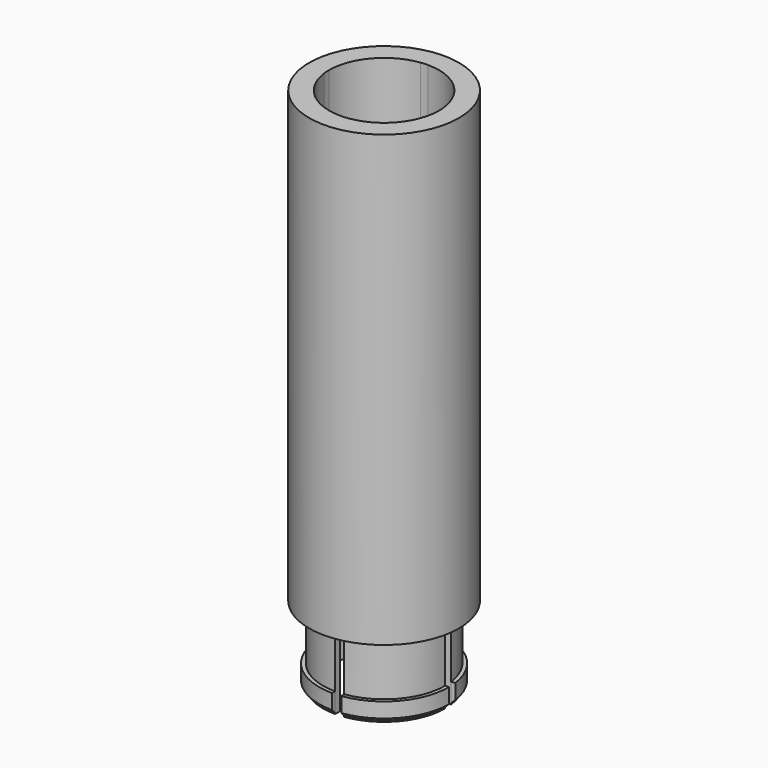
from build123d import *
from build123d import SkipClean  # not in build123d's __all__

# Parameters (mm, degrees)
F0_R          = 15
F1_DEPTH      = 90
F2_DEPTH      = 15
F3_START      = -11
F3_DEPTH      = 4
F4_T2_ANGLE   = 105.003910896
F4_2_T2_ANGLE = 105.003910896
F4_3_T2_ANGLE = 105.003910896
F4_4_T2_ANGLE = 105.003910896


# Not quite as in the source:
# - a fillet or chamfer that OpenCascade refuses, or shapes differently, is made with other operations: its cross-section is extruded or revolved along the edge and cut away or added


with BuildPart() as f1:
    # F0 (on Top) → F1 (new body)
    with BuildSketch(Plane.XY):
        with Locations((-39.9452038109, 28.1051583588)):
            Circle(F0_R)
        with BuildLine():
            ThreePointArc((-27.061585061, 29.8407758013), (-26.9743317556, 28.9749158684), (-26.9452038109, 28.1051583588))
            ThreePointArc((-26.9452038109, 28.1051583588), (-30.1584007897, 19.5483782036), (-38.2095863684, 15.2215396089))
            ThreePointArc((-38.2095863684, 15.2215396089), (-39.0754463013, 15.1342863035), (-39.9452038109, 15.1051583588))
            ThreePointArc((-39.9452038109, 15.1051583588), (-48.5019839661, 18.3183553376), (-52.8288225609, 26.3695409163))
            ThreePointArc((-52.8288225609, 26.3695409163), (-52.9160758662, 27.2354008492), (-52.9452038109, 28.1051583588))
            ThreePointArc((-52.9452038109, 28.1051583588), (-49.7320068322, 36.661938514), (-41.6808212534, 40.9887771087))
            ThreePointArc((-41.6808212534, 40.9887771087), (-40.8149613205, 41.0760304141), (-39.9452038109, 41.1051583588))
            ThreePointArc((-39.9452038109, 41.1051583588), (-31.3884236558, 37.89196138), (-27.061585061, 29.8407758013))
        make_face(mode=Mode.SUBTRACT)
        with BuildLine():
            ThreePointArc((-52.0855368637, 26.4696726918), (-48.0083235725, 18.8829785888), (-39.9452038109, 15.8551583588))
            Line((-39.9452038109, 15.8551583588), (-39.9452038109, 17.1051583588))
            ThreePointArc((-39.9452038109, 17.1051583588), (-47.1855562499, 19.8240173409), (-50.8467273686, 26.6365589844))
            Line((-50.8467273686, 26.6365589844), (-52.0855368637, 26.4696726918))
        make_face()
        with BuildLine():
            ThreePointArc((-27.8048707581, 29.7406440258), (-27.7226512973, 28.9247375506), (-27.6952038109, 28.1051583588))
            Line((-27.6952038109, 28.1051583588), (-26.9452038109, 28.1051583588))
            ThreePointArc((-26.9452038109, 28.1051583588), (-26.9743317556, 28.9749158684), (-27.061585061, 29.8407758013))
            Line((-27.061585061, 29.8407758013), (-27.8048707581, 29.7406440258))
        make_face()
        with BuildLine():
            ThreePointArc((-39.9452038109, 40.3551583588), (-31.8820840493, 37.3273381288), (-27.8048707581, 29.7406440258))
            Line((-27.8048707581, 29.7406440258), (-27.061585061, 29.8407758013))
            ThreePointArc((-27.061585061, 29.8407758013), (-31.3884236558, 37.89196138), (-39.9452038109, 41.1051583588))
            Line((-39.9452038109, 41.1051583588), (-39.9452038109, 40.3551583588))
        make_face()
        with BuildLine():
            ThreePointArc((-41.5806894779, 40.2454914116), (-40.7647830027, 40.3277108724), (-39.9452038109, 40.3551583588))
            Line((-39.9452038109, 40.3551583588), (-39.9452038109, 41.1051583588))
            ThreePointArc((-39.9452038109, 41.1051583588), (-40.8149613205, 41.0760304141), (-41.6808212534, 40.9887771087))
            Line((-41.6808212534, 40.9887771087), (-41.5806894779, 40.2454914116))
        make_face()
        with BuildLine():
            ThreePointArc((-52.1952038109, 28.1051583588), (-49.1673835809, 36.1682781204), (-41.5806894779, 40.2454914116))
            Line((-41.5806894779, 40.2454914116), (-41.6808212534, 40.9887771087))
            ThreePointArc((-41.6808212534, 40.9887771087), (-49.7320068322, 36.661938514), (-52.9452038109, 28.1051583588))
            Line((-52.9452038109, 28.1051583588), (-52.1952038109, 28.1051583588))
        make_face()
        with BuildLine():
            Line((-52.8288225609, 26.3695409163), (-52.0855368637, 26.4696726918))
            ThreePointArc((-52.0855368637, 26.4696726918), (-52.1677563246, 27.2855791671), (-52.1952038109, 28.1051583588))
            Line((-52.1952038109, 28.1051583588), (-52.9452038109, 28.1051583588))
            ThreePointArc((-52.9452038109, 28.1051583588), (-52.9160758662, 27.2354008492), (-52.8288225609, 26.3695409163))
        make_face()
        with BuildLine():
            Line((-39.9452038109, 15.1051583588), (-39.9452038109, 15.8551583588))
            ThreePointArc((-39.9452038109, 15.8551583588), (-48.0083235725, 18.8829785888), (-52.0855368637, 26.4696726918))
            Line((-52.0855368637, 26.4696726918), (-52.8288225609, 26.3695409163))
            ThreePointArc((-52.8288225609, 26.3695409163), (-48.5019839661, 18.3183553376), (-39.9452038109, 15.1051583588))
        make_face()
        with BuildLine():
            Line((-38.2095863684, 15.2215396089), (-38.309718144, 15.964825306))
            ThreePointArc((-38.309718144, 15.964825306), (-39.1256246192, 15.8826058452), (-39.9452038109, 15.8551583588))
            Line((-39.9452038109, 15.8551583588), (-39.9452038109, 15.1051583588))
            ThreePointArc((-39.9452038109, 15.1051583588), (-39.0754463013, 15.1342863035), (-38.2095863684, 15.2215396089))
        make_face()
        with BuildLine():
            Line((-26.9452038109, 28.1051583588), (-27.6952038109, 28.1051583588))
            ThreePointArc((-27.6952038109, 28.1051583588), (-30.7230240409, 20.0420385972), (-38.309718144, 15.964825306))
            Line((-38.309718144, 15.964825306), (-38.2095863684, 15.2215396089))
            ThreePointArc((-38.2095863684, 15.2215396089), (-30.1584007897, 19.5483782036), (-26.9452038109, 28.1051583588))
        make_face()
        with BuildLine():
            ThreePointArc((-38.309718144, 15.964825306), (-30.7230240409, 20.0420385972), (-27.6952038109, 28.1051583588))
            Line((-27.6952038109, 28.1051583588), (-28.9452038109, 28.1051583588))
            ThreePointArc((-28.9452038109, 28.1051583588), (-31.664062793, 20.8648059198), (-38.4766044365, 17.2036348012))
            Line((-38.4766044365, 17.2036348012), (-38.309718144, 15.964825306))
        make_face()
        with BuildLine():
            Line((-29.0436802533, 29.5737577332), (-27.8048707581, 29.7406440258))
            ThreePointArc((-27.8048707581, 29.7406440258), (-31.8820840493, 37.3273381288), (-39.9452038109, 40.3551583588))
            Line((-39.9452038109, 40.3551583588), (-39.9452038109, 39.1051583588))
            ThreePointArc((-39.9452038109, 39.1051583588), (-32.7048513719, 36.3862993768), (-29.0436802533, 29.5737577332))
        make_face()
        with BuildLine():
            Line((-41.4138031853, 39.0066819164), (-41.5806894779, 40.2454914116))
            ThreePointArc((-41.5806894779, 40.2454914116), (-49.1673835809, 36.1682781204), (-52.1952038109, 28.1051583588))
            Line((-52.1952038109, 28.1051583588), (-50.9452038109, 28.1051583588))
            ThreePointArc((-50.9452038109, 28.1051583588), (-48.2263448289, 35.3455107978), (-41.4138031853, 39.0066819164))
        make_face()
        with BuildLine():
            Line((-39.9452038109, 39.1051583588), (-39.9452038109, 40.3551583588))
            ThreePointArc((-39.9452038109, 40.3551583588), (-40.7647830027, 40.3277108724), (-41.5806894779, 40.2454914116))
            Line((-41.5806894779, 40.2454914116), (-41.4138031853, 39.0066819164))
            ThreePointArc((-41.4138031853, 39.0066819164), (-40.6811524729, 39.0805116364), (-39.9452038109, 39.1051583588))
        make_face()
        with BuildLine():
            Line((-28.9452038109, 28.1051583588), (-27.6952038109, 28.1051583588))
            ThreePointArc((-27.6952038109, 28.1051583588), (-27.7226512973, 28.9247375506), (-27.8048707581, 29.7406440258))
            Line((-27.8048707581, 29.7406440258), (-29.0436802533, 29.5737577332))
            ThreePointArc((-29.0436802533, 29.5737577332), (-28.9698505334, 28.8411070208), (-28.9452038109, 28.1051583588))
        make_face()
        with BuildLine():
            ThreePointArc((-39.9452038109, 15.8551583588), (-39.1256246192, 15.8826058452), (-38.309718144, 15.964825306))
            Line((-38.309718144, 15.964825306), (-38.4766044365, 17.2036348012))
            ThreePointArc((-38.4766044365, 17.2036348012), (-39.209255149, 17.1298050813), (-39.9452038109, 17.1051583588))
            Line((-39.9452038109, 17.1051583588), (-39.9452038109, 15.8551583588))
        make_face()
        with BuildLine():
            ThreePointArc((-52.1952038109, 28.1051583588), (-52.1677563246, 27.2855791671), (-52.0855368637, 26.4696726918))
            Line((-52.0855368637, 26.4696726918), (-50.8467273686, 26.6365589844))
            ThreePointArc((-50.8467273686, 26.6365589844), (-50.9205570885, 27.3692096968), (-50.9452038109, 28.1051583588))
            Line((-50.9452038109, 28.1051583588), (-52.1952038109, 28.1051583588))
        make_face()
    extrude(amount=F1_DEPTH)

    # F0 (on Top) → F2 (join)
    with BuildSketch(Plane.XY):
        with BuildLine():
            Line((-41.4138031853, 39.0066819164), (-41.5806894779, 40.2454914116))
            ThreePointArc((-41.5806894779, 40.2454914116), (-49.1673835809, 36.1682781204), (-52.1952038109, 28.1051583588))
            Line((-52.1952038109, 28.1051583588), (-50.9452038109, 28.1051583588))
            ThreePointArc((-50.9452038109, 28.1051583588), (-48.2263448289, 35.3455107978), (-41.4138031853, 39.0066819164))
        make_face()
        with BuildLine():
            Line((-29.0436802533, 29.5737577332), (-27.8048707581, 29.7406440258))
            ThreePointArc((-27.8048707581, 29.7406440258), (-31.8820840493, 37.3273381288), (-39.9452038109, 40.3551583588))
            Line((-39.9452038109, 40.3551583588), (-39.9452038109, 39.1051583588))
            ThreePointArc((-39.9452038109, 39.1051583588), (-32.7048513719, 36.3862993768), (-29.0436802533, 29.5737577332))
        make_face()
        with BuildLine():
            ThreePointArc((-38.309718144, 15.964825306), (-30.7230240409, 20.0420385972), (-27.6952038109, 28.1051583588))
            Line((-27.6952038109, 28.1051583588), (-28.9452038109, 28.1051583588))
            ThreePointArc((-28.9452038109, 28.1051583588), (-31.664062793, 20.8648059198), (-38.4766044365, 17.2036348012))
            Line((-38.4766044365, 17.2036348012), (-38.309718144, 15.964825306))
        make_face()
        with BuildLine():
            ThreePointArc((-52.0855368637, 26.4696726918), (-48.0083235725, 18.8829785888), (-39.9452038109, 15.8551583588))
            Line((-39.9452038109, 15.8551583588), (-39.9452038109, 17.1051583588))
            ThreePointArc((-39.9452038109, 17.1051583588), (-47.1855562499, 19.8240173409), (-50.8467273686, 26.6365589844))
            Line((-50.8467273686, 26.6365589844), (-52.0855368637, 26.4696726918))
        make_face()
    with SkipClean():  # cleaning this boolean's faces spoils the solid; the shape is the same uncleaned
        extrude(amount=-F2_DEPTH)


with BuildPart() as f3:
    # F0 (on Top) → F3 (new body)
    with BuildSketch(Plane.XY.offset(F3_START)):
        with BuildLine():
            ThreePointArc((-39.9452038109, 40.3551583588), (-31.8820840493, 37.3273381288), (-27.8048707581, 29.7406440258))
            Line((-27.8048707581, 29.7406440258), (-27.061585061, 29.8407758013))
            ThreePointArc((-27.061585061, 29.8407758013), (-31.3884236558, 37.89196138), (-39.9452038109, 41.1051583588))
            Line((-39.9452038109, 41.1051583588), (-39.9452038109, 40.3551583588))
        make_face()
    extrude(amount=-F3_DEPTH)

    # F4#4: chamfer of 1 on 1 edges, made by hand

    # F4_4_s1 → F4_4_t2 (revolve, cut)
    with BuildSketch(Plane(origin=(1.6299605955, 25.4415695588, 0), x_dir=(0, 0, 1), z_dir=(-0.0639357458, -0.9979540172, 0))):
        Polygon((-14, 28.6604008708), (-15, 29.6604008708), (-15, 28.6604008708), align=None)
    revolve(axis=Axis((-39.9452038109, 28.1051583588, -15), (0, 0, 1)), revolution_arc=F4_4_T2_ANGLE, mode=Mode.SUBTRACT)


with BuildPart() as f3b:
    # F0 (on Top) → F3, piece 2 (new body)
    with BuildSketch(Plane.XY.offset(F3_START)):
        with BuildLine():
            Line((-39.9452038109, 15.1051583588), (-39.9452038109, 15.8551583588))
            ThreePointArc((-39.9452038109, 15.8551583588), (-48.0083235725, 18.8829785888), (-52.0855368637, 26.4696726918))
            Line((-52.0855368637, 26.4696726918), (-52.8288225609, 26.3695409163))
            ThreePointArc((-52.8288225609, 26.3695409163), (-48.5019839661, 18.3183553376), (-39.9452038109, 15.1051583588))
        make_face()
    extrude(amount=-F3_DEPTH)

    # F4#3: chamfer of 1 on 1 edges, made by hand

    # F4_3_s1 → F4_3_t2 (revolve, cut)
    with BuildSketch(Plane(origin=(1.6299605955, 25.4415695588, 0), x_dir=(0, 0, 1), z_dir=(0.0639357458, 0.9979540172, 0))):
        Polygon((-14, -54.6604008708), (-15, -53.6604008708), (-15, -54.6604008708), align=None)
    revolve(axis=Axis((-39.9452038109, 28.1051583588, -15), (0, 0, 1)), revolution_arc=F4_3_T2_ANGLE, mode=Mode.SUBTRACT)


with BuildPart() as f3c:
    # F0 (on Top) → F3, piece 3 (new body)
    with BuildSketch(Plane.XY.offset(F3_START)):
        with BuildLine():
            Line((-26.9452038109, 28.1051583588), (-27.6952038109, 28.1051583588))
            ThreePointArc((-27.6952038109, 28.1051583588), (-30.7230240409, 20.0420385972), (-38.309718144, 15.964825306))
            Line((-38.309718144, 15.964825306), (-38.2095863684, 15.2215396089))
            ThreePointArc((-38.2095863684, 15.2215396089), (-30.1584007897, 19.5483782036), (-26.9452038109, 28.1051583588))
        make_face()
    extrude(amount=-F3_DEPTH)

    # F4: chamfer of 1 on 1 edges, made by hand

    # F4_s1 → F4_t2 (revolve, cut)
    with BuildSketch(Plane(origin=(-41.5751644064, 2.6635888001, 0), x_dir=(0, 0, 1), z_dir=(-0.9979540172, 0.0639357458, 0))):
        Polygon((-14, 12.4937292909), (-15, 13.4937292909), (-15, 12.4937292909), align=None)
    revolve(axis=Axis((-39.9452038109, 28.1051583588, -15), (0, 0, 1)), revolution_arc=F4_T2_ANGLE, mode=Mode.SUBTRACT)


with BuildPart() as f3d:
    # F0 (on Top) → F3, piece 4 (new body)
    with BuildSketch(Plane.XY.offset(F3_START)):
        with BuildLine():
            ThreePointArc((-52.1952038109, 28.1051583588), (-49.1673835809, 36.1682781204), (-41.5806894779, 40.2454914116))
            Line((-41.5806894779, 40.2454914116), (-41.6808212534, 40.9887771087))
            ThreePointArc((-41.6808212534, 40.9887771087), (-49.7320068322, 36.661938514), (-52.9452038109, 28.1051583588))
            Line((-52.9452038109, 28.1051583588), (-52.1952038109, 28.1051583588))
        make_face()
    extrude(amount=-F3_DEPTH)

    # F4#2: chamfer of 1 on 1 edges, made by hand

    # F4_2_s1 → F4_2_t2 (revolve, cut)
    with BuildSketch(Plane(origin=(-41.5751644064, 2.6635888001, 0), x_dir=(0, 0, 1), z_dir=(0.9979540172, -0.0639357458, 0))):
        Polygon((-14, -38.4937292909), (-15, -37.4937292909), (-15, -38.4937292909), align=None)
    revolve(axis=Axis((-39.9452038109, 28.1051583588, -15), (0, 0, 1)), revolution_arc=F4_2_T2_ANGLE, mode=Mode.SUBTRACT)


solid = Compound([f1.part, f3.part, f3b.part, f3c.part, f3d.part])
